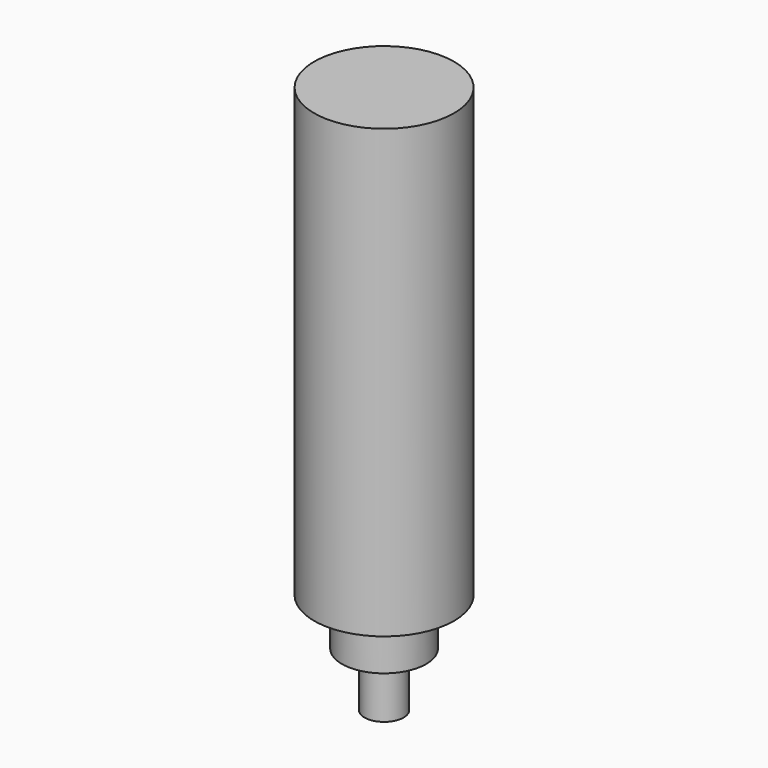
from build123d import *


# Not quite as in the source:
# - a feature names something its author has since deleted; it is built from what else it names


with BuildPart() as f1:
    # F0 (on Front) → F1 (revolve)
    with BuildSketch(Plane.XZ):
        Polygon((71.4, -228.2), (71.4, 0), (35.7, 0), (35.7, -280), (45.7, -280), (45.7, -252.2), (57.2, -252.2), (57.2, -228.2), align=None)
    revolve(axis=Axis((35.7, 0, -140), (0, 0, -1)))


solid = f1.part
